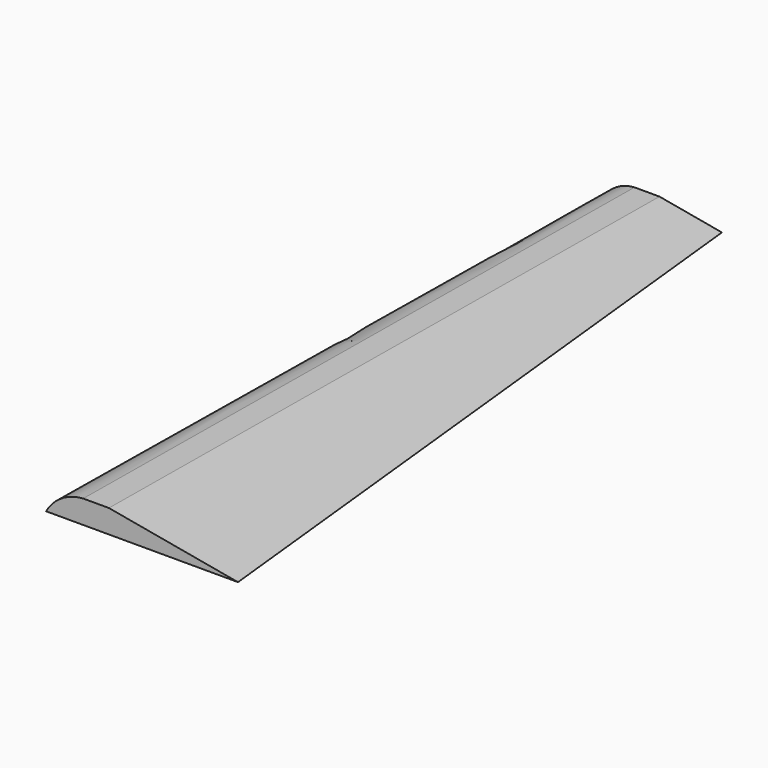
from build123d import *

# Parameters (mm, degrees)
F1_DEPTH               = 1100
DRAFT_F1_DRAFTED_ANGLE = -0.5


# Not quite as in the source:
# - an extrude with a draft is written as a straight extrude whose walls are then drafted


with BuildPart() as f1:
    # F0 (on Front) → F1 (new body)
    with BuildSketch(Plane.XZ):
        with BuildLine():
            ThreePointArc((40.3481945395, 18), (18.5428946305, 12.656448968), (0, 0))
            Line((0, 0), (180, 0))
            Line((180, 0), (80.26804775, 18))
            Line((80.26804775, 18), (40.3481945395, 18))
        make_face()
    extrude(amount=F1_DEPTH)

    # draft_F1_drafted
    draft_f1_drafted_walls = [f1.faces().sort_by_distance(p)[0] for p in [
        (90, -733.3333333333, 0),
        (130.134023875, -733.3333333333, 9),
        (60.3081211448, -733.3333333333, 18),
        (18.5428946305, -733.3333333333, 12.656448968),
    ]]
    draft(draft_f1_drafted_walls, neutral_plane=Plane.XZ, angle=DRAFT_F1_DRAFTED_ANGLE)


solid = f1.part
